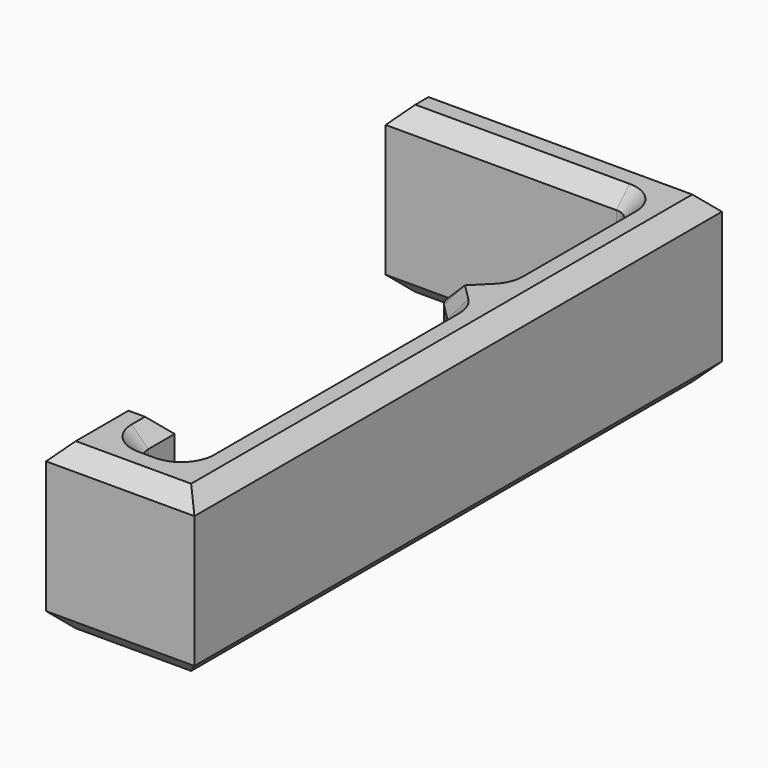
from build123d import *

# Parameters (mm, degrees)
F1_DEPTH = 10
F2_R     = 1
F3_SIZE  = 0.99999


# Not quite as in the source:
# - a fillet or chamfer is up to 0.001 mm smaller than in the source, because OpenCascade refuses the exact size


with BuildPart() as f1:
    # F0 (on Top) → F1 (new body)
    with BuildSketch(Plane.XY):
        Polygon((18, 0), (0, 0), (0, -3), (15, -3), (15, -13), (13, -15), (15, -17), (15, -37), (12, -37), (12, -34), (9, -34), (9, -40), (18, -40), align=None)
    extrude(amount=F1_DEPTH)

    # F2
    f2_edges = [f1.edges().sort_by_distance(p)[0] for p in [
        (13, -15, 5),
        (15, -13, 5),
        (15, -37, 5),
        (15, -17, 5),
        (15, -3, 5),
        (12, -37, 5),
    ]]
    fillet(f2_edges, radius=F2_R)

    # F3 (size 1 in the source; OpenCascade refuses exactly that, so slightly less here)
    f3_edges = [f1.edges().sort_by_distance(p)[0] for p in [
        (7, -3, 10),
        (14.707107, -3.292893, 10),
        (0, -1.5, 10),
        (15, -8.292893, 10),
        (9, 0, 10),
        (14.92388, -12.96847, 10),
        (18, -20, 10),
        (14.207107, -13.792893, 10),
        (13.5, -40, 10),
        (13.414214, -15, 10),
        (9, -37, 10),
        (14.207107, -16.207107, 10),
        (10.5, -34, 10),
        (14.92388, -17.03153, 10),
        (12, -35, 10),
        (15, -26.707107, 10),
        (12.292893, -36.707107, 10),
        (14.707107, -36.707107, 10),
        (13.5, -37, 10),
        (7, -3, 0),
        (14.707107, -3.292893, 0),
        (0, -1.5, 0),
        (15, -8.292893, 0),
        (9, 0, 0),
        (14.92388, -12.96847, 0),
        (18, -20, 0),
        (14.207107, -13.792893, 0),
        (13.5, -40, 0),
        (13.414214, -15, 0),
        (9, -37, 0),
        (14.207107, -16.207107, 0),
        (10.5, -34, 0),
        (14.92388, -17.03153, 0),
        (12, -35, 0),
        (15, -26.707107, 0),
        (12.292893, -36.707107, 0),
        (14.707107, -36.707107, 0),
        (13.5, -37, 0),
    ]]
    chamfer(f3_edges, length=F3_SIZE)


solid = f1.part
